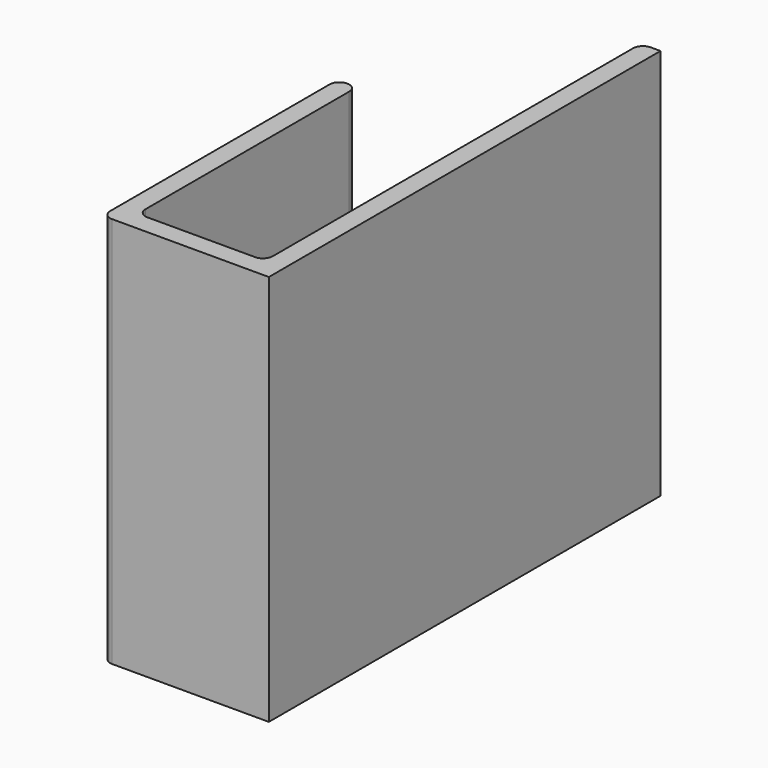
from build123d import *

# Parameters (mm, degrees)
F0_W     = 13
F0_H     = 2
F1_DEPTH = 40
F2_R     = 0.99999


# Not quite as in the source:
# - a fillet or chamfer is up to 0.001 mm smaller than in the source, because OpenCascade refuses the exact size


with BuildPart() as f1:
    # F0 (on Top) → F1 (new body)
    with BuildSketch(Plane.XY):
        Polygon((-24.5838956386, 17.7643506003), (-26.5838956386, 17.7643506003), (-26.5838956386, -12.2356493997), (-24.5838956386, -12.2356493997), (-24.5838956386, -10.2356493997), align=None)
        with Locations((-18.0838956386, -11.2356493997)):
            Rectangle(F0_W, F0_H)
        Polygon((-11.5838956386, 37.7643506003), (-11.5838956386, -10.2356493997), (-11.5838956386, -12.2356493997), (-9.5838956386, -12.2356493997), (-9.5838956386, 37.7643506003), align=None)
    extrude(amount=F1_DEPTH)

    # F2 (radius 1 in the source; OpenCascade refuses exactly that, so slightly less here)
    f2_edges = [f1.edges().sort_by_distance(p)[0] for p in [
        (-26.583896, 17.764351, 20),
        (-24.583896, 17.764351, 20),
        (-11.583896, 37.764351, 20),
        (-26.583896, -12.235649, 20),
        (-24.583896, -10.235649, 20),
        (-11.583896, -10.235649, 20),
    ]]
    fillet(f2_edges, radius=F2_R)


solid = f1.part
